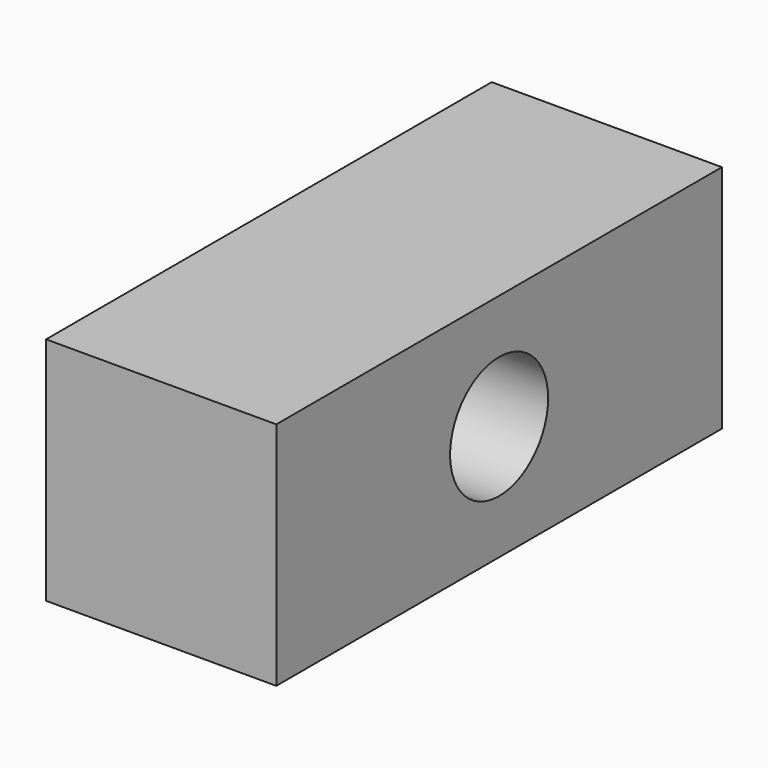
from build123d import *

# Parameters (mm, degrees)
F0_W     = 6.2
F0_H     = 6.2
F1_DEPTH = 15
F2_R     = 1.65
F3_DEPTH = 6.2


# Not quite as in the source:
# - a feature names something its author has since deleted; it is built from what else it names


with BuildPart() as f1:
    # F0 (on Front) → F1 (new body)
    with BuildSketch(Plane.XZ):
        with Locations((22.738877362, -3.1)):
            Rectangle(F0_W, F0_H)
    extrude(amount=F1_DEPTH)

    # F2 (on face) → F3 (cut, through all)
    with BuildSketch(Plane.YZ.offset(25.838877362)):
        with Locations((-7.5, -3.1)):
            Circle(F2_R)
    extrude(amount=-F3_DEPTH, mode=Mode.SUBTRACT)


solid = f1.part
